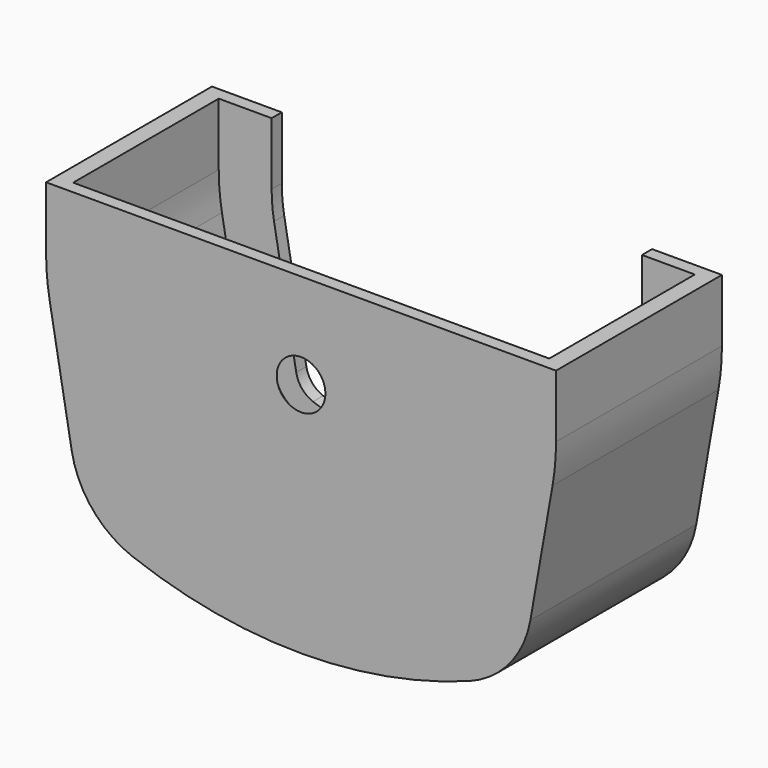
from build123d import *

# Parameters (mm, degrees)
F1_DEPTH = 17.2
F2_R     = 1.5
F3_DEPTH = 1.2
F5_DEPTH = 1.2


# Not quite as in the source:
# - a fillet or chamfer that OpenCascade refuses, or shapes differently, is made with other operations: its cross-section is extruded or revolved along the edge and cut away or added


with BuildPart() as f1:
    # F0 (on Front) → F1 (new body)
    with BuildSketch(Plane.XZ):
        with BuildLine():
            Line((-20.1, 5.7260450742), (-22.1961550602, 17.6139311585))
            ThreePointArc((-22.1961550602, 17.6139311585), (-22.4238939618, 19.3437798569), (-22.5, 21.0868947118))
            Line((-22.5, 21.0868947118), (-22.5, 27))
            Line((-22.5, 27), (-24.1, 27))
            Line((-24.1, 27), (-24.1, 21.0868947118))
            ThreePointArc((-24.1, 21.0868947118), (-24.0178054788, 19.2043306685), (-23.7718474651, 17.3360940742))
            Line((-23.7718474651, 17.3360940742), (-21.6756924048, 5.44820799))
            ThreePointArc((-21.6756924048, 5.44820799), (-19.7066672631, 1.205023255), (-15.889887542, -1.4993933668))
            ThreePointArc((-15.889887542, -1.4993933668), (0, -4.3622248316), (15.889887542, -1.4993933668))
            ThreePointArc((15.889887542, -1.4993933668), (19.7066672631, 1.205023255), (21.6756924048, 5.44820799))
            Line((21.6756924048, 5.44820799), (23.7718474651, 17.3360940742))
            ThreePointArc((23.7718474651, 17.3360940742), (24.0178054788, 19.2043306685), (24.1, 21.0868947118))
            Line((24.1, 21.0868947118), (24.1, 27))
            Line((24.1, 27), (22.5, 27))
            Line((22.5, 27), (22.5, 21.0868947118))
            ThreePointArc((22.5, 21.0868947118), (22.4238939618, 19.3437798569), (22.1961550602, 17.6139311585))
            Line((22.1961550602, 17.6139311585), (20.1, 5.7260450742))
            ThreePointArc((20.1, 5.7260450742), (18.477177081, 2.2289147982), (15.3314795087, 0))
            ThreePointArc((15.3314795087, 0), (0, -2.7622248316), (-15.3314795087, 0))
            ThreePointArc((-15.3314795087, 0), (-18.477177081, 2.2289147982), (-20.1, 5.7260450742))
        make_face()
    extrude(amount=F1_DEPTH)

    # F2 (on face) → F3 (join)
    with BuildSketch(Plane.XZ.offset(17.2)):
        with BuildLine():
            Line((24.1, 27), (-24.1, 27))
            Line((-24.1, 27), (-24.1, 21.0868947118))
            ThreePointArc((-24.1, 21.0868947118), (-24.0178054788, 19.2043306685), (-23.7718474651, 17.3360940742))
            Line((-23.7718474651, 17.3360940742), (-21.6756924048, 5.44820799))
            ThreePointArc((-21.6756924048, 5.44820799), (-19.7066672631, 1.205023255), (-15.889887542, -1.4993933668))
            ThreePointArc((-15.889887542, -1.4993933668), (0, -4.3622248316), (15.889887542, -1.4993933668))
            ThreePointArc((15.889887542, -1.4993933668), (19.7066672631, 1.205023255), (21.6756924048, 5.44820799))
            Line((21.6756924048, 5.44820799), (23.7718474651, 17.3360940742))
            ThreePointArc((23.7718474651, 17.3360940742), (24.0178054788, 19.2043306685), (24.1, 21.0868947118))
            Line((24.1, 21.0868947118), (24.1, 27))
        make_face()
        with Locations((0, 18)):
            Circle(F2_R, mode=Mode.SUBTRACT)
    extrude(amount=F3_DEPTH)

    # F4 (on face) → F5 (join)
    with BuildSketch(Plane(origin=(0, 0, 0), x_dir=(-1, 0, 0), z_dir=(0, 1, 0))):
        with BuildLine():
            Line((-24.1, 27), (-24.1, 21.0868947118))
            ThreePointArc((-24.1, 21.0868947118), (-24.0178054788, 19.2043306685), (-23.7718474651, 17.3360940742))
            Line((-23.7718474651, 17.3360940742), (-21.6756924048, 5.44820799))
            ThreePointArc((-21.6756924048, 5.44820799), (-19.7066672631, 1.205023255), (-15.889887542, -1.4993933668))
            ThreePointArc((-15.889887542, -1.4993933668), (0, -4.3622248316), (15.889887542, -1.4993933668))
            ThreePointArc((15.889887542, -1.4993933668), (19.7066672631, 1.205023255), (21.6756924048, 5.44820799))
            Line((21.6756924048, 5.44820799), (23.7718474651, 17.3360940742))
            ThreePointArc((23.7718474651, 17.3360940742), (24.0178054788, 19.2043306685), (24.1, 21.0868947118))
            Line((24.1, 21.0868947118), (24.1, 27))
            Line((24.1, 27), (17.5, 27))
            Line((17.5, 27), (17.5, 21.0868947118))
            ThreePointArc((17.5, 21.0868947118), (17.4429204714, 19.7795585706), (17.2721162952, 18.4821720468))
            Line((17.2721162952, 18.4821720468), (15.1759612349, 6.5942859626))
            ThreePointArc((15.1759612349, 6.5942859626), (14.6350202619, 5.4285758705), (13.5864544045, 4.6856042711))
            ThreePointArc((13.5864544045, 4.6856042711), (0, 2.2377751684), (-13.5864544045, 4.6856042711))
            ThreePointArc((-13.5864544045, 4.6856042711), (-14.6350202619, 5.4285758705), (-15.1759612349, 6.5942859626))
            Line((-15.1759612349, 6.5942859626), (-17.2721162952, 18.4821720468))
            ThreePointArc((-17.2721162952, 18.4821720468), (-17.4429204714, 19.7795585706), (-17.5, 21.0868947118))
            Line((-17.5, 21.0868947118), (-17.5, 27))
            Line((-17.5, 27), (-24.1, 27))
        make_face()
    extrude(amount=F5_DEPTH)

    # F6: chamfer of 2 on 1 edges, made by hand

    # F6_s1 → F6_t2 (revolve, cut)
    with BuildSketch(Plane.XY.offset(18)):
        Polygon((3.5, -17.2), (1.5, -19.2), (1.5, -17.2), align=None)
    revolve(axis=Axis((0, -17.2, 18), (0, -1, 0)), mode=Mode.SUBTRACT)


solid = f1.part
